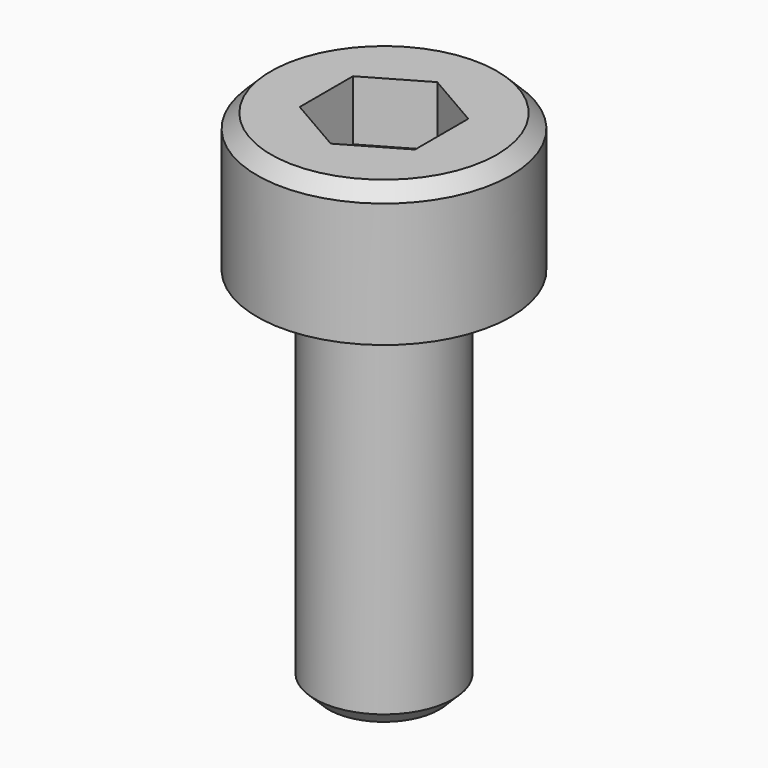
from build123d import *

# Parameters (mm, degrees)
F2_R      = 1.5
F3_DEPTH  = 8
F2_R_2    = 2.75
F3_FACE_R = 1.5
F4_DEPTH  = 3
F5_SIZE   = 0.3
F7_DEPTH  = 1.3


with BuildPart() as f3:
    # F2 (on Top) → F3 (new body)
    with BuildSketch(Plane.XY):
        Circle(F2_R)
    extrude(amount=-F3_DEPTH)

    # F2 (on Top) + F3_face (on face) → F4 (join)
    with BuildSketch(Plane.XY):
        Circle(F2_R_2)
        Circle(F2_R, mode=Mode.SUBTRACT)
    with BuildSketch(Plane.XY):
        Circle(F3_FACE_R)
    extrude(amount=F4_DEPTH)

    # F5
    f5_edges = [f3.edges().sort_by_distance(p)[0] for p in [
        (-1.5, 0, -8),
        (-2.75, 0, 3),
    ]]
    chamfer(f5_edges, length=F5_SIZE)

    # F6 (on face) → F7 (cut)
    with BuildSketch(Plane.XY.offset(3)):
        Polygon((1.25, -0.7216878365), (1.25, 0.7216878365), (0, 1.443375673), (-1.25, 0.7216878365), (-1.25, -0.7216878365), (0, -1.443375673), align=None)
    extrude(amount=-F7_DEPTH, mode=Mode.SUBTRACT)


solid = f3.part
